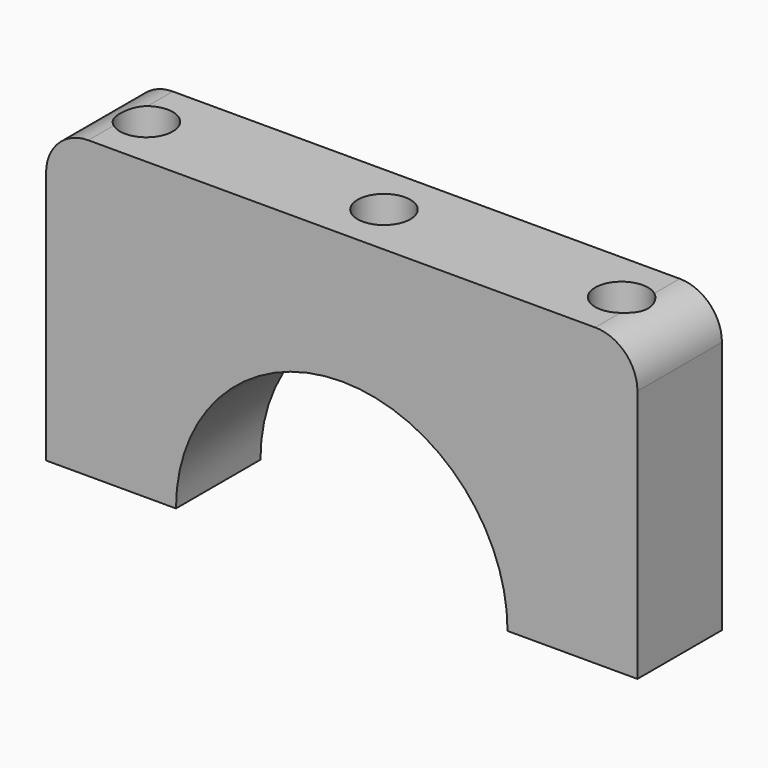
from build123d import *

# Parameters (mm, degrees)
F1_DEPTH    = 12.7
F2_R        = 3.175
F3_DEPTH    = 35.561
F4_R        = 3.175
F5_DEPTH    = 15.8764097817
F6_T1_DEPTH = 38.1


# Not quite as in the source:
# - a fillet or chamfer that OpenCascade refuses, or shapes differently, is made with other operations: its cross-section is extruded or revolved along the edge and cut away or added


with BuildPart() as f1:
    # F0 (on Front) → F1 (new body)
    with BuildSketch(Plane.XZ):
        with BuildLine():
            Line((0, 35.56), (0, 0))
            Line((0, 0), (15.621, 0))
            ThreePointArc((15.621, 0), (35.56, 19.939), (55.499, 0))
            Line((55.499, 0), (71.12, 0))
            Line((71.12, 0), (71.12, 35.56))
            Line((71.12, 35.56), (0, 35.56))
        make_face()
    extrude(amount=F1_DEPTH)

    # F2 (on face) → F3 (cut, through all)
    with BuildSketch(Plane.XY.offset(35.56)):
        with Locations((6.985, -6.35)):
            Circle(F2_R)
        with Locations((64.135, -6.35)):
            Circle(F2_R)
    extrude(amount=-F3_DEPTH, mode=Mode.SUBTRACT)

    # F4 (on face) → F5 (cut, through all)
    with BuildSketch(Plane.XY.offset(35.56)):
        with Locations((35.56, -6.35)):
            Circle(F4_R)
    extrude(amount=-F5_DEPTH, mode=Mode.SUBTRACT)

    # F6: fillet of radius 5.08 on 2 edges, made by hand

    # F6_s2 → F6_t1 (cut)
    with BuildSketch(Plane.XZ.offset(-12.7)):
        with BuildLine():
            ThreePointArc((0, 30.48), (1.4878975516, 34.0721024484), (5.08, 35.56))
            Line((5.08, 35.56), (0, 35.56))
            Line((0, 35.56), (0, 30.48))
        make_face()
        with BuildLine():
            ThreePointArc((66.04, 35.56), (69.6321024484, 34.0721024484), (71.12, 30.48))
            Line((71.12, 30.48), (71.12, 35.56))
            Line((71.12, 35.56), (66.04, 35.56))
        make_face()
    extrude(amount=F6_T1_DEPTH, mode=Mode.SUBTRACT)


solid = f1.part
